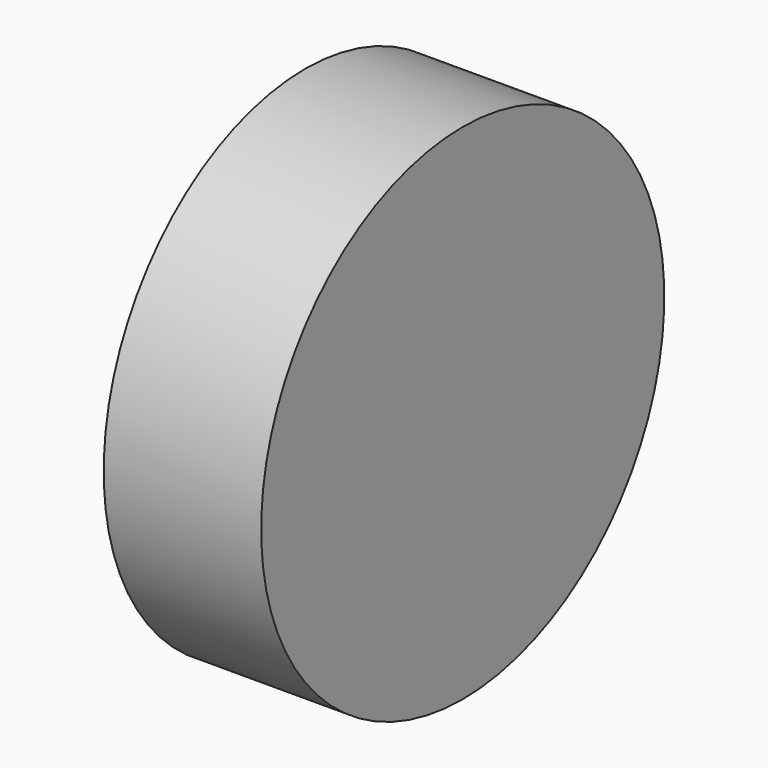
from build123d import *

# Parameters (mm, degrees)
F2_DEPTH = 25.4


# Not quite as in the source:
# - a feature of the source that left no trace in its solid (it failed there, or was rolled back) is left out


with BuildPart() as f1:
    # F0 (on Front) → F1 (revolve)
    with BuildSketch(Plane.XZ):
        with BuildLine():
            Line((-15.24, 0), (0, 0))
            Line((0, 0), (0, 50.8))
            Line((0, 50.8), (-6.35, 50.8))
            Line((-6.35, 50.8), (-4.7617064118, 41.792339449))
            ThreePointArc((-4.7617064118, 41.792339449), (-4.8311637627, 41.5331210865), (-5.0743828734, 41.4197061526))
            Line((-5.0743828734, 41.4197061526), (-6.2835011077, 41.4197061526))
            ThreePointArc((-6.2835011077, 41.4197061526), (-6.5080075107, 41.3267125556), (-6.6010011077, 41.1022061526))
            Line((-6.6010011077, 41.1022061526), (-6.6010011077, 40.4672061526))
            ThreePointArc((-6.6010011077, 40.4672061526), (-6.5080075107, 40.2426997495), (-6.2835011077, 40.1497061526))
            Line((-6.2835011077, 40.1497061526), (-5.0743828734, 40.1497061526))
            ThreePointArc((-5.0743828734, 40.1497061526), (-4.8311637627, 40.0362912186), (-4.7617064118, 39.7770728561))
            Line((-4.7617064118, 39.7770728561), (-5.2010717431, 37.2853082403))
            ThreePointArc((-5.2010717431, 37.2853082403), (-5.3096631386, 37.0972224261), (-5.5137482047, 37.0229415367))
            Line((-5.5137482047, 37.0229415367), (-6.8348340718, 37.0229415367))
            ThreePointArc((-6.8348340718, 37.0229415367), (-7.0593404748, 36.9299479398), (-7.1523340718, 36.7054415367))
            Line((-7.1523340718, 36.7054415367), (-7.1523340718, 36.0704415367))
            ThreePointArc((-7.1523340718, 36.0704415367), (-7.2453276688, 35.8459351337), (-7.4698340718, 35.7529415367))
            Line((-7.4698340718, 35.7529415367), (-8.7398340718, 35.7529415367))
            ThreePointArc((-8.7398340718, 35.7529415367), (-8.9643404748, 35.6599479398), (-9.0573340718, 35.4354415367))
            Line((-9.0573340718, 35.4354415367), (-9.0573340718, 34.8004415367))
            ThreePointArc((-9.0573340718, 34.8004415367), (-8.9643404748, 34.5759351337), (-8.7398340718, 34.4829415367))
            Line((-8.7398340718, 34.4829415367), (-3.5686493249, 34.4829415367))
            ThreePointArc((-3.5686493249, 34.4829415367), (-3.3254302142, 34.3695266028), (-3.2559728633, 34.1103082403))
            Line((-3.2559728633, 34.1103082403), (-7.113602572, 12.2326030065))
            ThreePointArc((-7.113602572, 12.2326030065), (-7.2221939675, 12.0445171922), (-7.4262790336, 11.9702363029))
            Line((-7.4262790336, 11.9702363029), (-8.1123649007, 11.9702363029))
            ThreePointArc((-8.1123649007, 11.9702363029), (-8.3368713037, 11.8772427059), (-8.4298649007, 11.6527363029))
            Line((-8.4298649007, 11.6527363029), (-8.4298649007, 8.9432889844))
            ThreePointArc((-8.4298649007, 8.9432889844), (-8.4596121783, 8.8091076862), (-8.5432798346, 8.7000698737))
            Line((-8.5432798346, 8.7000698737), (-15.1265850661, 3.176020882))
            ThreePointArc((-15.1265850661, 3.176020882), (-15.2102527224, 3.0669830694), (-15.24, 2.9328017713))
            Line((-15.24, 2.9328017713), (-15.24, 0))
        make_face()
    revolve(axis=Axis((-7.62, 0, 0), (-1, 0, 0)))

    # F2 (add): a face of the model
    f2_faces = [f1.faces().sort_by_distance(p)[0] for p in [
        (0, 0, 0),
    ]]
    extrude(f2_faces, amount=F2_DEPTH)


solid = f1.part
